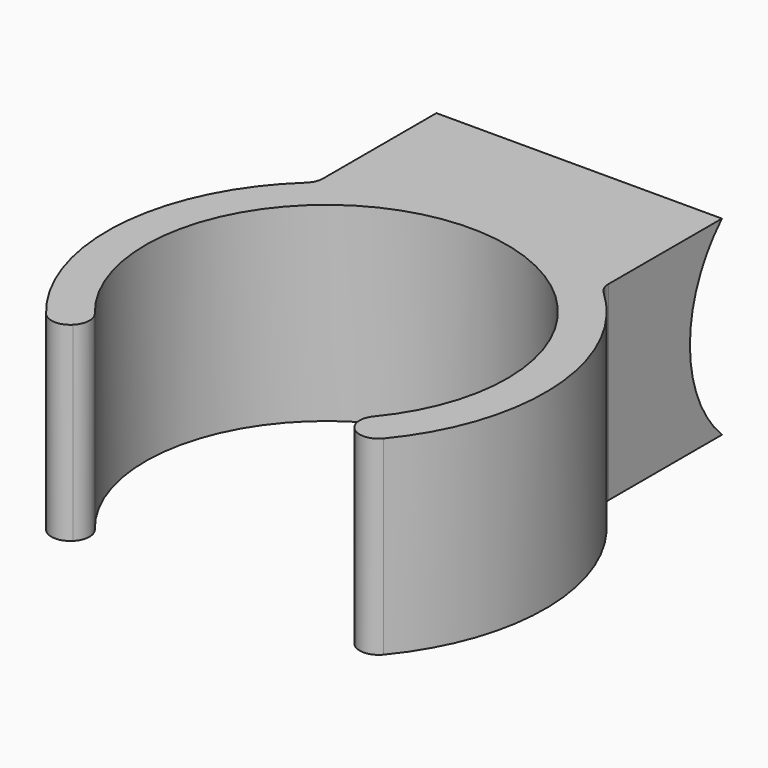
from build123d import *

# Parameters (mm, degrees)
F1_DEPTH = 10
F3_DEPTH = 15
F4_R     = 0.99999


# Not quite as in the source:
# - a fillet or chamfer is up to 0.001 mm smaller than in the source, because OpenCascade refuses the exact size


with BuildPart() as f1:
    # F0 (on Top) → F1 (new body)
    with BuildSketch(Plane.XY):
        with BuildLine():
            ThreePointArc((-6.7175144213, -6.7175144213), (0, 9.5), (6.7175144213, -6.7175144213))
            Line((6.7175144213, -6.7175144213), (8.1317279836, -8.1317279836))
            ThreePointArc((8.1317279836, -8.1317279836), (11.4919258811, 0.430859077), (7.5, 8.7177978871))
            Line((7.5, 8.7177978871), (7.5, 9.5))
            Line((7.5, 9.5), (7.5, 14.5))
            Line((7.5, 14.5), (-7.5, 14.5))
            Line((-7.5, 14.5), (-7.5, 9.5))
            Line((-7.5, 9.5), (-7.5, 8.7177978871))
            ThreePointArc((-7.5, 8.7177978871), (-11.4919258811, 0.430859077), (-8.1317279836, -8.1317279836))
            Line((-8.1317279836, -8.1317279836), (-6.7175144213, -6.7175144213))
        make_face()
    extrude(amount=F1_DEPTH)

    # F2 (on face) → F3 (join, through all)
    with BuildSketch(Plane.YZ.offset(7.5)):
        with BuildLine():
            ThreePointArc((14.5, 5), (15.0465956117, 7.7117470016), (16.6010205144, 10))
            Line((16.6010205144, 10), (14.5, 10))
            Line((14.5, 10), (14.5, 5))
        make_face()
        with BuildLine():
            Line((14.5, 0), (16.6010205144, 0))
            ThreePointArc((16.6010205144, 0), (15.0465956117, 2.2882529984), (14.5, 5))
            Line((14.5, 5), (14.5, 0))
        make_face()
    extrude(amount=-F3_DEPTH)

    # F4 (radius 1 in the source; OpenCascade refuses exactly that, so slightly less here)
    f4_edges = [f1.edges().sort_by_distance(p)[0] for p in [
        (-6.717514, -6.717514, 5),
        (-8.131728, -8.131728, 5),
        (8.131728, -8.131728, 5),
        (6.717514, -6.717514, 5),
        (7.5, 8.717798, 5),
        (-7.5, 8.717798, 5),
    ]]
    fillet(f4_edges, radius=F4_R)


solid = f1.part
